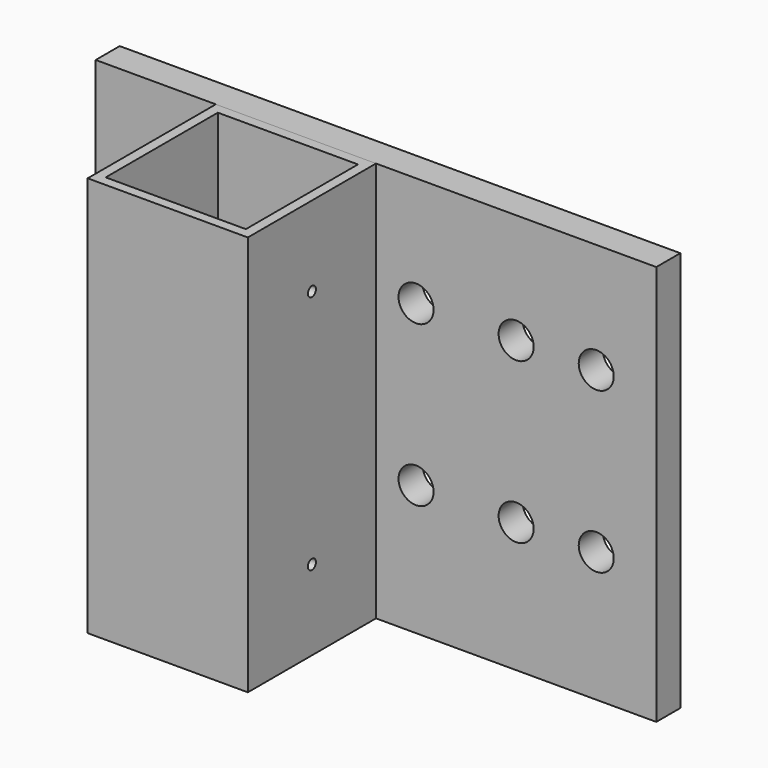
from build123d import *

# Parameters (mm, degrees)
F0_W     = 177.8
F0_H     = 127
F1_DEPTH = 9.525
F3_D     = 11.1125
F4_W     = 50.8
F4_H     = 50.8
F4_W_2   = 44.45
F4_H_2   = 44.45
F5_DEPTH = 127
F7_D     = 3.175
F8_W     = 22.225
F8_H     = 44.45
F9_DEPTH = 3.175
F10_D    = 6.35


# Not quite as in the source:
# - a feature names something its author has since deleted; it is built from what else it names


with BuildPart() as f1:
    # F0 (on Front) → F1 (new body)
    with BuildSketch(Plane.XZ):
        with Locations((88.9, 63.5)):
            Rectangle(F0_W, F0_H)
    extrude(amount=-F1_DEPTH)

    # F3 (through all)
    with Locations(Plane.XZ):
        with Locations((101.6, 92.075), (133.35, 92.075), (158.75, 92.075), (158.75, 41.275), (133.35, 41.275), (101.6, 41.275), (19.05, 92.075), (19.05, 41.275)):
            Hole(F3_D / 2)


with BuildPart() as f5:
    # F4 (on face) → F5 (new body)
    with BuildSketch(Plane.XY.offset(127)):
        with Locations((63.5, -25.4)):
            Rectangle(F4_W, F4_H)
        with Locations((63.5, -25.4)):
            Rectangle(F4_W_2, F4_H_2, mode=Mode.SUBTRACT)
    extrude(amount=-F5_DEPTH)

    # F7 (through all)
    with Locations(Plane(origin=(38.1, 0, 0), x_dir=(0, -1, 0), z_dir=(-1, 0, 0))):
        with Locations((25.4, 101.6), (25.4, 25.4)):
            Hole(F7_D / 2)

    # F8 (on face) → F9 (join)
    with BuildSketch(Plane(origin=(0, 0, 0), x_dir=(1, 0, 0), z_dir=(0, 0, -1))):
        with Locations((74.6125, 25.4)):
            Rectangle(F8_W, F8_H)
        with Locations((52.3875, 25.4)):
            Rectangle(F8_W, F8_H)
    extrude(amount=-F9_DEPTH)

    # F10 (through all)
    with Locations(Plane(origin=(0, 0, 0), x_dir=(1, 0, 0), z_dir=(0, 0, -1))):
        with Locations((63.5, 25.4)):
            Hole(F10_D / 2)


solid = Compound([f1.part, f5.part])
